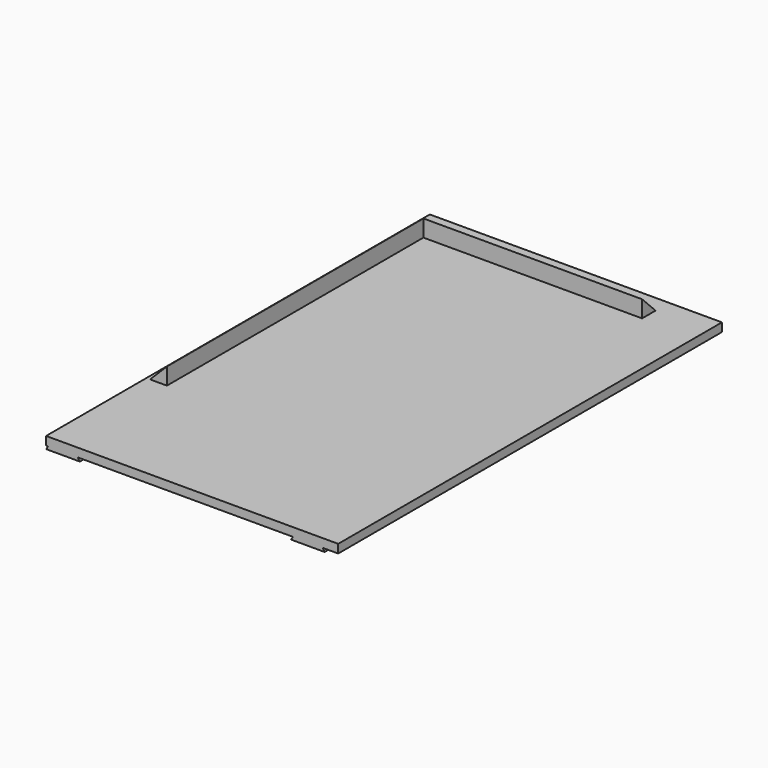
from build123d import *

# Parameters (mm, degrees)
F0_W      = 96.52
F0_H      = 2.54
F1_DEPTH  = 142.24
F2_W      = 10
F2_H      = 142.24
F3_DEPTH  = 0.9017
F5_DEPTH  = 142.241
F8_DEPTH  = 5
F9_SIZE   = 4.99999
F10_W     = 9.9
F10_H     = 142.24
F11_DEPTH = 3.4427


# Not quite as in the source:
# - a fillet or chamfer is up to 0.001 mm smaller than in the source, because OpenCascade refuses the exact size


with BuildPart() as f1:
    # F0 (on Front) → F1 (new body)
    with BuildSketch(Plane.XZ):
        with Locations((-48.26, 1.27)):
            Rectangle(F0_W, F0_H)
    extrude(amount=F1_DEPTH)

    # F2 (on face) → F3 (join)
    with BuildSketch(Plane(origin=(0, 0, 0), x_dir=(1, 0, 0), z_dir=(0, 0, -1))):
        with Locations((-81.614, 71.12)):
            Rectangle(F2_W, F2_H)
        with Locations((-9.0132, 71.12)):
            Rectangle(F2_W, F2_H)
    extrude(amount=F3_DEPTH)

    # F4 (on face) → F5 (cut, through all)
    with BuildSketch(Plane.XZ.offset(142.24)):
        Polygon((-86.614, 0), (-86.614, -0.9017), (-86.0057956704, 0), align=None)
        Polygon((-77.2222043296, 0), (-76.614, -0.9017), (-76.614, 0), align=None)
        Polygon((-14.0132, 0), (-14.0132, -0.9017), (-13.4049956704, 0), align=None)
        Polygon((-4.6214043296, 0), (-4.0132, -0.9017), (-4.0132, 0), align=None)
    extrude(amount=-F5_DEPTH, mode=Mode.SUBTRACT)

    # F7 (on face) → F8 (join)
    with BuildSketch(Plane.XY.offset(2.54)):
        Polygon((-15.67, -5), (-85.52, -5), (-85.52, -105.076), (-80.52, -105.076), (-80.52, -10), (-15.67, -10), align=None)
    extrude(amount=F8_DEPTH)

    # F9 (size 5 in the source; OpenCascade refuses exactly that, so slightly less here)
    f9_edges = [f1.edges().sort_by_distance(p)[0] for p in [
        (-85.52, -55.038, 7.54),
        (-50.595, -5, 7.54),
    ]]
    chamfer(f9_edges, length=F9_SIZE)

    # F10 (on face) → F11 (cut, through all)
    with BuildSketch(Plane.XY.offset(2.54)):
        with Locations((-91.57, -71.12)):
            Rectangle(F10_W, F10_H)
    extrude(amount=-F11_DEPTH, mode=Mode.SUBTRACT)


solid = f1.part
